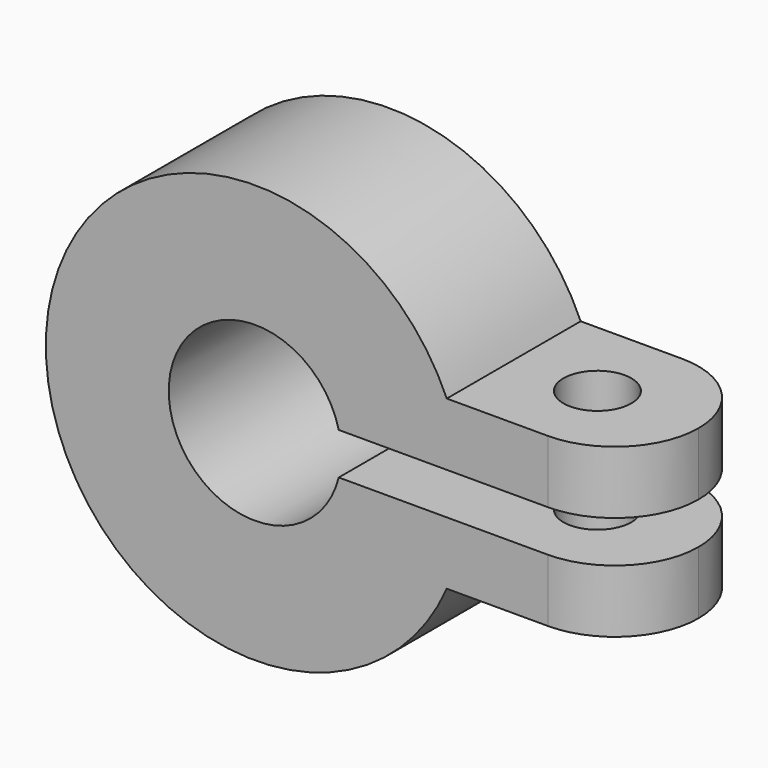
from build123d import *

# Parameters (mm, degrees)
F1_DEPTH = 8
F2_R     = 1.625
F3_DEPTH = 14.001
F4_R     = 3.99999


# Not quite as in the source:
# - a fillet or chamfer is up to 0.001 mm smaller than in the source, because OpenCascade refuses the exact size


with BuildPart() as f1:
    # F0 (on Front) → F1 (new body)
    with BuildSketch(Plane.XZ):
        with BuildLine():
            ThreePointArc((4.0019526484, -1), (-4.125, 0), (4.0019526484, 1))
            Line((4.0019526484, 1), (18, 1))
            Line((18, 1), (18, 4))
            Line((18, 4), (9.1651513899, 4))
            ThreePointArc((9.1651513899, 4), (-10, 0), (9.1651513899, -4))
            Line((9.1651513899, -4), (18, -4))
            Line((18, -4), (18, -1))
            Line((18, -1), (4.0019526484, -1))
        make_face()
    extrude(amount=F1_DEPTH)

    # F2 (on face) → F3 (cut, through all)
    with BuildSketch(Plane.XY.offset(4)):
        with Locations((13.1651513899, -4.0000034496)):
            Circle(F2_R)
    extrude(amount=-F3_DEPTH, mode=Mode.SUBTRACT)

    # F4 (radius 4 in the source; OpenCascade refuses exactly that, so slightly less here)
    f4_edges = [f1.edges().sort_by_distance(p)[0] for p in [
        (18, -8, 2.5),
        (18, -8, -2.5),
        (18, 0, -2.5),
        (18, 0, 2.5),
    ]]
    fillet(f4_edges, radius=F4_R)


solid = f1.part
